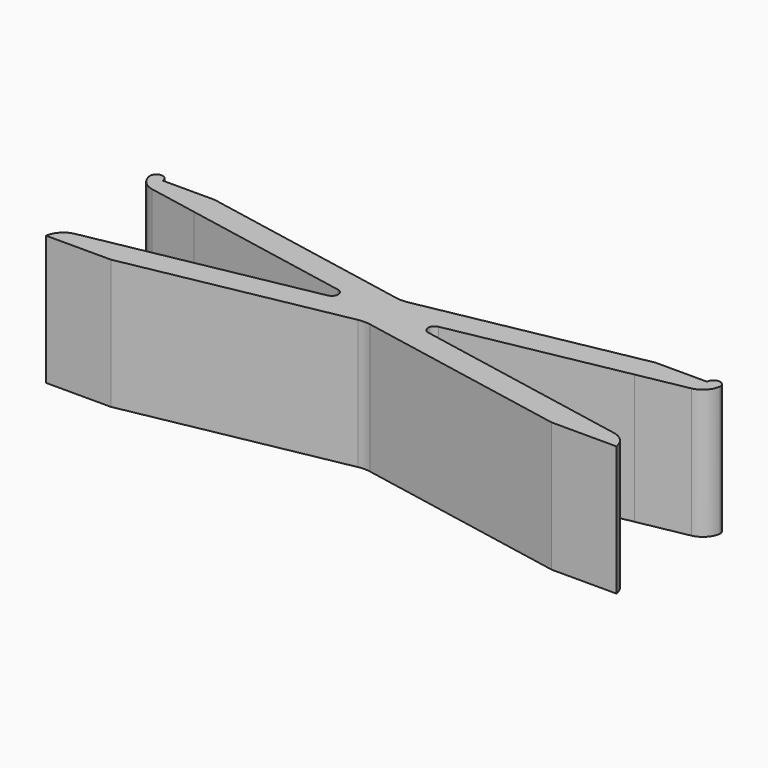
from build123d import *

# Parameters (mm, degrees)
F1_DEPTH    = 20
F2_T1_DEPTH = 20
F3_T1_DEPTH = 32.2692705553
F5_R        = 5


# Not quite as in the source:
# - a fillet or chamfer that OpenCascade refuses, or shapes differently, is made with other operations: its cross-section is extruded or revolved along the edge and cut away or added


with BuildPart() as f1:
    # F0 (on Top) → F1 (new body)
    with BuildSketch(Plane.XY):
        Polygon((0, 2.0882352941), (0, 0), (10, 0), (44, 6.5), (44, 13.5), (10, 20), (2, 20), (0, 20), (0, 17.9117647059), (10, 16), (41.3846153846, 10), (10, 4), align=None)
        with BuildLine():
            Line((0, 20), (2, 20))
            ThreePointArc((2, 20), (1, 21), (0, 20))
        make_face()
    extrude(amount=-F1_DEPTH)

    # F2: fillet of radius 1 on 1 edges, made by hand

    # F2_s2 → F2_t1 (join)
    with BuildSketch(Plane.XY.offset(-20)):
        with BuildLine():
            ThreePointArc((36.2468915209, 10.9822119151), (37.0591157136, 10), (36.2468915209, 9.0177880849))
            Line((36.2468915209, 9.0177880849), (41.3846153846, 10))
            Line((41.3846153846, 10), (36.2468915209, 10.9822119151))
        make_face()
    extrude(amount=F2_T1_DEPTH)

    # F3: fillet of radius 3 on 2 edges, made by hand

    # F3_s2 → F3_t1 (cut)
    with BuildSketch(Plane.XY.offset(-26.1346352777)):
        with BuildLine():
            ThreePointArc((0, 20), (0.7936912123, 18.3364871524), (2.4102047458, 17.4509902692))
            Line((2.4102047458, 17.4509902692), (2.3989381974, 17.3920575543))
            Line((2.3989381974, 17.3920575543), (-0.0112665484, 17.852831991))
            Line((-0.0112665484, 17.852831991), (-0.06, 17.9117647059))
            ThreePointArc((-0.06, 17.9117647059), (-0.06, 18.9558823529), (-0.0594706434, 19.9920474797))
            Line((-0.0594706434, 19.9920474797), (0, 20))
        make_face()
        with BuildLine():
            ThreePointArc((0, 0), (0.7936912123, 1.6635128476), (2.4102047458, 2.5490097308))
            Line((2.4102047458, 2.5490097308), (2.3989381974, 2.6079424457))
            Line((2.3989381974, 2.6079424457), (-0.0112665484, 2.147168009))
            Line((-0.0112665484, 2.147168009), (-0.06, 2.0882352941))
            ThreePointArc((-0.06, 2.0882352941), (-0.06, 1.0441176471), (-0.0594706434, 0.0079525203))
            Line((-0.0594706434, 0.0079525203), (0, 0))
        make_face()
    extrude(amount=F3_T1_DEPTH, mode=Mode.SUBTRACT)

    # F4: F1 across face


with BuildPart() as f1_1:
    add(f1.part)
    add(f1.part.mirror(Plane(origin=(44, 10, -10), x_dir=(0, 1, 0), z_dir=(1, 0, 0))))

    # F5
    f5_edges = [f1_1.edges().sort_by_distance(p)[0] for p in [
        (44, 13.5, -10),
        (44, 6.5, -10),
    ]]
    fillet(f5_edges, radius=F5_R)


solid = f1_1.part
